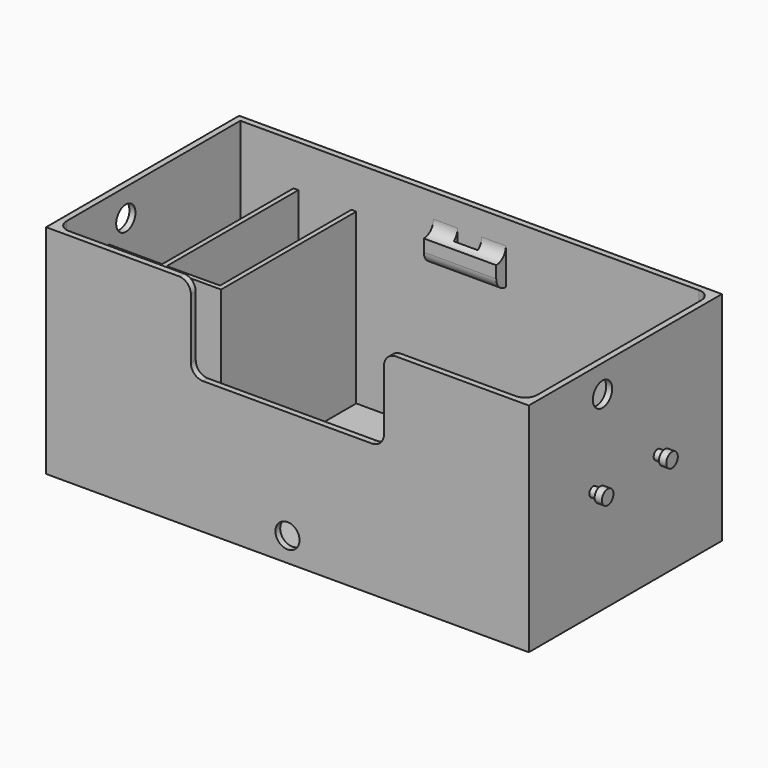
from build123d import *

# Parameters (mm, degrees)
F0_W          = 200
F0_H          = 100
F1_DEPTH      = 90
F2_T          = -2.5
F4_DEPTH      = 70
F5_W          = 80
F5_H          = 35
F5_R          = 5
F6_DEPTH      = 3
F8_DEPTH      = 3
F9_R          = 3.3
F10_DEPTH     = 1.5
F11_R         = 7.8
F12_DEPTH     = 3
F13_R         = 5
F14_R         = 5
F16_DEPTH     = 3
F17_R         = 2
F17_R_2       = 3
F18_R         = 3
F18_R_2       = 2
F19_DEPTH     = 3
F21_DEPTH     = 3
F22_R         = 3
F22_R_2       = 2
F23_DEPTH     = 3
F24_R         = 5
F25_DEPTH     = 400
F26_W         = 22
F26_H         = 30
F26_H_2       = 6.5
F27_W         = 21.9996754151
F27_H         = 30
F29_DEPTH     = 10
F31_W         = 15
F31_H         = 10
F32_DEPTH     = 5
F33_W         = 10
F33_H         = 2
F34_DEPTH     = 10
F35_T4_DEPTH  = 10
F35_T9_DEPTH  = 10
F35_T14_DEPTH = 22.5
F35_T21_DEPTH = 22.5
F35_T27_DEPTH = 22.5
F35_T33_DEPTH = 22.5
F35_T39_DEPTH = 22.5
F35_T45_DEPTH = 22.5
F35_T52_DEPTH = 10
F35_T57_DEPTH = 10
F35_T59_DEPTH = 55
F36_DEPTH     = 35


# Not quite as in the source:
# - a fillet or chamfer that OpenCascade refuses, or shapes differently, is made with other operations: its cross-section is extruded or revolved along the edge and cut away or added
# - ends of sketch curves that miss each other by under 0.0002 mm in the source are joined
# - a feature names something its author has since deleted; it is built from what else it names


with BuildPart() as f1:
    # F0 (on Top) → F1 (new body)
    with BuildSketch(Plane.XY):
        with Locations((-6.9181565195, -17.9440884142)):
            Rectangle(F0_W, F0_H)
    extrude(amount=F1_DEPTH)

    # F2
    f2_openings = [f1.faces().sort_by_distance(p)[0] for p in [
        (-6.918157, -17.944088, 90),
    ]]
    offset(amount=F2_T, openings=f2_openings)

    # F3 (on face) → F4 (join)
    with BuildSketch(Plane.XY.offset(2.5)):
        Polygon((-82.4181565195, -38.4440884142), (-104.4181565195, -38.4440884142), (-104.4181565195, -40.4440884142), (-82.4181565195, -40.4440884142), (-80.4181565195, -40.4440884142), (-80.4181565195, -38.6240089446), (-80.4181565195, 29.5559115858), (-82.4181565195, 29.5559115858), align=None)
        Polygon((-58.4188922454, -38.4440884142), (-80.4181565195, -38.6240089446), (-80.4181565195, -40.4440884142), (-56.4181565195, -40.4440884142), (-56.4181565195, -38.4440884142), (-56.4181565195, 29.5559115858), (-58.4181565195, 29.5559115858), align=None)
    extrude(amount=F4_DEPTH)

    # F5 (on face) → F6 (cut)
    with BuildSketch(Plane.XZ.offset(67.9440884142)):
        with Locations((-6.9181565195, 72.5)):
            Rectangle(F5_W, F5_H)
        with Locations((-6.9181565195, 10)):
            Circle(F5_R)
    extrude(amount=-F6_DEPTH, mode=Mode.SUBTRACT)

    # F7 (on face) → F8 (cut)
    with BuildSketch(Plane(origin=(0, 0, 0), x_dir=(1, 0, 0), z_dir=(0, 0, -1))):
        with BuildLine():
            ThreePointArc((-3.6181565195, 17.9440884142), (-4.5847041416, 20.2775407921), (-6.9181565195, 21.2440884142))
            Line((-6.9181565195, 21.2440884142), (-6.9181565195, 14.6440884142))
            ThreePointArc((-6.9181565195, 14.6440884142), (-4.5847041416, 15.6106360363), (-3.6181565195, 17.9440884142))
        make_face()
        with BuildLine():
            Line((-6.9181565195, 14.6440884142), (-6.9181565195, 21.2440884142))
            ThreePointArc((-6.9181565195, 21.2440884142), (-10.2181565195, 17.9440884142), (-6.9181565195, 14.6440884142))
        make_face()
    extrude(amount=-F8_DEPTH, mode=Mode.SUBTRACT)

    # F9 (on face) → F10 (cut)
    with BuildSketch(Plane.XY.offset(2.5)):
        Polygon((-4.1346192375, -12.3481595191), (-10.3726044595, -12.735509968), (-13.1561417415, -18.3314388632), (-9.7016938016, -23.5400173094), (-3.4637085796, -23.1526668604), (-0.6801712975, -17.5567379653), align=None)
        with Locations((-6.9181565195, -17.9440884142)):
            Circle(F9_R, mode=Mode.SUBTRACT)
    extrude(amount=-F10_DEPTH, mode=Mode.SUBTRACT)

    # F11 (on face) → F12 (cut)
    with BuildSketch(Plane(origin=(0, 32.0559115858, 0), x_dir=(-1, 0, 0), z_dir=(0, 1, 0))):
        with Locations((6.9181565195, 18.6942107975)):
            Circle(F11_R)
    extrude(amount=-F12_DEPTH, mode=Mode.SUBTRACT)

    # F13
    f13_edges = [f1.edges().sort_by_distance(p)[0] for p in [
        (90.581843, 29.555912, 46.25),
        (90.581843, -65.444088, 46.25),
        (-104.418157, -65.444088, 46.25),
    ]]
    fillet(f13_edges, radius=F13_R)

    # F14
    f14_edges = [f1.edges().sort_by_distance(p)[0] for p in [
        (33.081843, -66.694088, 55),
        (-46.918157, -66.694088, 55),
        (-46.918157, -66.694088, 90),
        (33.081843, -66.694088, 90),
    ]]
    fillet(f14_edges, radius=F14_R)

    # F15 (on face) → F16 (join)
    with BuildSketch(Plane.YZ.offset(93.0818434805)):
        with BuildLine():
            ThreePointArc((-32.6107550809, 45), (-34.6107550809, 47), (-36.6107550809, 45))
            Line((-36.6107550809, 45), (-34.6107550809, 45))
            Line((-34.6107550809, 45), (-32.6107550809, 45))
        make_face()
        with BuildLine():
            ThreePointArc((0.7225782525, 45), (-1.2774217475, 47), (-3.2774217475, 45))
            Line((-3.2774217475, 45), (-1.2774217475, 45))
            Line((-1.2774217475, 45), (0.7225782525, 45))
        make_face()
        with BuildLine():
            Line((-1.2774217475, 45), (-3.2774217475, 45))
            ThreePointArc((-3.2774217475, 45), (-1.2774217475, 43), (0.7225782525, 45))
            Line((0.7225782525, 45), (-1.2774217475, 45))
        make_face()
        with BuildLine():
            Line((-34.6107550809, 45), (-36.6107550809, 45))
            ThreePointArc((-36.6107550809, 45), (-34.6107550809, 43), (-32.6107550809, 45))
            Line((-32.6107550809, 45), (-34.6107550809, 45))
        make_face()
    extrude(amount=F16_DEPTH)

    # F17 (on face) + F18 (on face) → F19 (join)
    with BuildSketch(Plane.YZ.offset(96.0818434805)):
        with Locations((-34.6107550809, 45)):
            Circle(F17_R)
        with Locations((-1.2774217475, 45)):
            Circle(F17_R_2)
    with BuildSketch(Plane.YZ.offset(96.0818434805)):
        with Locations((-34.6107550809, 45)):
            Circle(F18_R)
        with Locations((-34.6107550809, 45)):
            Circle(F18_R_2, mode=Mode.SUBTRACT)
    extrude(amount=F19_DEPTH)

    # F20 (on face) → F21 (join)
    with BuildSketch(Plane(origin=(-106.9181565195, 0, 0), x_dir=(0, -1, 0), z_dir=(-1, 0, 0))):
        with BuildLine():
            ThreePointArc((3.2774217475, 45), (1.2774217475, 47), (-0.7225782525, 45))
            Line((-0.7225782525, 45), (1.2774217475, 45))
            Line((1.2774217475, 45), (3.2774217475, 45))
        make_face()
        with BuildLine():
            Line((1.2774217475, 45), (-0.7225782525, 45))
            ThreePointArc((-0.7225782525, 45), (1.2774217475, 43), (3.2774217475, 45))
            Line((3.2774217475, 45), (1.2774217475, 45))
        make_face()
        with BuildLine():
            ThreePointArc((36.6107550809, 45), (34.6107550809, 47), (32.6107550809, 45))
            Line((32.6107550809, 45), (34.6107550809, 45))
            Line((34.6107550809, 45), (36.6107550809, 45))
        make_face()
        with BuildLine():
            Line((34.6107550809, 45), (32.6107550809, 45))
            ThreePointArc((32.6107550809, 45), (34.6107550809, 43), (36.6107550809, 45))
            Line((36.6107550809, 45), (34.6107550809, 45))
        make_face()
    extrude(amount=F21_DEPTH)

    # F22 (on face) → F23 (join)
    with BuildSketch(Plane(origin=(-109.9181565195, 0, 0), x_dir=(0, -1, 0), z_dir=(-1, 0, 0))):
        with Locations((1.2774217475, 45)):
            Circle(F22_R)
        with Locations((1.2774217475, 45)):
            Circle(F22_R_2, mode=Mode.SUBTRACT)
        with Locations((1.2774217475, 45)):
            Circle(F22_R_2)
        with Locations((34.6107550809, 45)):
            Circle(F22_R)
    extrude(amount=F23_DEPTH)

    # F24 (on face) → F25 (cut, symmetric)
    with BuildSketch(Plane.YZ.offset(-104.4181565195)):
        with Locations((-29.7736749053, 78.6124244332)):
            Circle(F24_R)
    extrude(amount=F25_DEPTH, both=True, mode=Mode.SUBTRACT)

    # F26 (on face) + F27 (on face) + F28 (on face) → F29 (join)
    with BuildSketch(Plane.XY.offset(2.5)):
        with Locations((-93.4181565195, 14.5559115858)):
            Rectangle(F26_W, F26_H)
        with Locations((-93.4181565195, -35.1940884142)):
            Rectangle(F26_W, F26_H_2)
    with BuildSketch(Plane.XY.offset(2.5)):
        with Locations((-69.418318812, 14.5559115858)):
            Rectangle(F27_W, F27_H)
        Polygon((-58.4181565195, 29.5559115858), (-58.4184811045, 29.5559115858), (-58.4184811045, -0.4440884142), align=None)
    with BuildSketch(Plane.XY.offset(2.5)):
        Polygon((-80.4181565195, -32.1240089446), (-80.4181565195, -38.6240089446), (-58.4188922454, -38.4440884142), (-58.4188238653, -32.1240089446), align=None)
    extrude(amount=F29_DEPTH)

    # F31 (on face) → F32 (join)
    with BuildSketch(Plane.XZ.offset(-29.5559115858)):
        with Locations((-16.9181565195, 70.1089176536)):
            Rectangle(F31_W, F31_H)
        with Locations((-1.9181565195, 70.1089176536)):
            Rectangle(F31_W, F31_H)
    extrude(amount=F32_DEPTH)

    # F33 (on face) → F34 (cut)
    with BuildSketch(Plane.XY.offset(75.1089176536)):
        with Locations((-9.4181565195, 28.5559115858)):
            Rectangle(F33_W, F33_H)
    extrude(amount=-F34_DEPTH, mode=Mode.SUBTRACT)

    # F35: fillet of radius 5 on 3 edges, made by hand


with BuildPart() as f35_tool2:
    # F35_s3 → F35_t4 (new body)
    with BuildSketch(Plane.YZ.offset(5.5818434805)):
        with BuildLine():
            ThreePointArc((29.5559115858, 80.1089176536), (28.0914454917, 76.5733837476), (24.5559115858, 75.1089176536))
            Line((24.5559115858, 75.1089176536), (29.5559115858, 75.1089176536))
            Line((29.5559115858, 75.1089176536), (29.5559115858, 80.1089176536))
        make_face()
    extrude(amount=-F35_T4_DEPTH)

    split(bisect_by=Plane.XZ.offset(-27.5559115858), keep=Keep.BOTTOM)


with BuildPart() as f1_1:
    add(f1.part)

    # F35_t1: union F35_tool2
    add(f35_tool2.part)


with BuildPart() as f35_tool7:
    # F35_s8 → F35_t9 (new body)
    with BuildSketch(Plane.YZ.offset(5.5818434805)):
        with BuildLine():
            ThreePointArc((29.5559115858, 80.1089176536), (28.0914454917, 76.5733837476), (24.5559115858, 75.1089176536))
            Line((24.5559115858, 75.1089176536), (29.5559115858, 75.1089176536))
            Line((29.5559115858, 75.1089176536), (29.5559115858, 80.1089176536))
        make_face()
    extrude(amount=-F35_T9_DEPTH)

    split(bisect_by=Plane.XZ.offset(-27.5559115858), keep=Keep.TOP)


with BuildPart() as f1_2:
    add(f1_1.part)

    # F35_t6: union F35_tool7
    add(f35_tool7.part)


with BuildPart() as f35_tool12:
    # F35_s13 → F35_t14 (new body)
    with BuildSketch(Plane.YZ.offset(5.5818434805)):
        with BuildLine():
            ThreePointArc((29.5559115858, 80.1089176536), (28.0914454917, 76.5733837476), (24.5559115858, 75.1089176536))
            Line((24.5559115858, 75.1089176536), (29.5559115858, 75.1089176536))
            Line((29.5559115858, 75.1089176536), (29.5559115858, 80.1089176536))
        make_face()
    extrude(amount=-F35_T14_DEPTH)

    split(bisect_by=Plane.YZ.offset(-4.4181565195), keep=Keep.BOTTOM)

    split(bisect_by=Plane.XZ.offset(-27.5559115858), keep=Keep.TOP)

    split(bisect_by=Plane.YZ.offset(-14.4181565195), keep=Keep.TOP)


with BuildPart() as f1_3:
    add(f1_2.part)

    # F35_t11: union F35_tool12
    add(f35_tool12.part)


with BuildPart() as f35_tool19:
    # F35_s20 → F35_t21 (new body)
    with BuildSketch(Plane.YZ.offset(5.5818434805)):
        with BuildLine():
            ThreePointArc((29.5559115858, 80.1089176536), (28.0914454917, 76.5733837476), (24.5559115858, 75.1089176536))
            Line((24.5559115858, 75.1089176536), (29.5559115858, 75.1089176536))
            Line((29.5559115858, 75.1089176536), (29.5559115858, 80.1089176536))
        make_face()
    extrude(amount=-F35_T21_DEPTH)

    split(bisect_by=Plane.XZ.offset(-27.5559115858), keep=Keep.BOTTOM)

    split(bisect_by=Plane.YZ.offset(-14.4181565195), keep=Keep.BOTTOM)


with BuildPart() as f1_4:
    add(f1_3.part)

    # F35_t18: union F35_tool19
    add(f35_tool19.part)


with BuildPart() as f35_tool25:
    # F35_s26 → F35_t27 (new body)
    with BuildSketch(Plane.YZ.offset(5.5818434805)):
        with BuildLine():
            ThreePointArc((29.5559115858, 80.1089176536), (28.0914454917, 76.5733837476), (24.5559115858, 75.1089176536))
            Line((24.5559115858, 75.1089176536), (29.5559115858, 75.1089176536))
            Line((29.5559115858, 75.1089176536), (29.5559115858, 80.1089176536))
        make_face()
    extrude(amount=-F35_T27_DEPTH)

    split(bisect_by=Plane.XZ.offset(-27.5559115858), keep=Keep.TOP)

    split(bisect_by=Plane.YZ.offset(-14.4181565195), keep=Keep.BOTTOM)


with BuildPart() as f1_5:
    add(f1_4.part)

    # F35_t24: union F35_tool25
    add(f35_tool25.part)


with BuildPart() as f35_tool31:
    # F35_s32 → F35_t33 (new body)
    with BuildSketch(Plane.YZ.offset(-1.9181565195)):
        with BuildLine():
            ThreePointArc((29.5559115858, 80.1089176536), (28.0914454917, 76.5733837476), (24.5559115858, 75.1089176536))
            Line((24.5559115858, 75.1089176536), (29.5559115858, 75.1089176536))
            Line((29.5559115858, 75.1089176536), (29.5559115858, 80.1089176536))
        make_face()
    extrude(amount=-F35_T33_DEPTH)

    split(bisect_by=Plane.YZ.offset(-4.4181565195), keep=Keep.TOP)

    split(bisect_by=Plane.XZ.offset(-27.5559115858), keep=Keep.BOTTOM)


with BuildPart() as f1_6:
    add(f1_5.part)

    # F35_t30: union F35_tool31
    add(f35_tool31.part)


with BuildPart() as f35_tool37:
    # F35_s38 → F35_t39 (new body)
    with BuildSketch(Plane.YZ.offset(-1.9181565195)):
        with BuildLine():
            ThreePointArc((29.5559115858, 80.1089176536), (28.0914454917, 76.5733837476), (24.5559115858, 75.1089176536))
            Line((24.5559115858, 75.1089176536), (29.5559115858, 75.1089176536))
            Line((29.5559115858, 75.1089176536), (29.5559115858, 80.1089176536))
        make_face()
    extrude(amount=-F35_T39_DEPTH)

    split(bisect_by=Plane.YZ.offset(-4.4181565195), keep=Keep.TOP)

    split(bisect_by=Plane.XZ.offset(-27.5559115858), keep=Keep.TOP)


with BuildPart() as f1_7:
    add(f1_6.part)

    # F35_t36: union F35_tool37
    add(f35_tool37.part)


with BuildPart() as f35_tool43:
    # F35_s44 → F35_t45 (new body)
    with BuildSketch(Plane.YZ.offset(-1.9181565195)):
        with BuildLine():
            ThreePointArc((29.5559115858, 80.1089176536), (28.0914454917, 76.5733837476), (24.5559115858, 75.1089176536))
            Line((24.5559115858, 75.1089176536), (29.5559115858, 75.1089176536))
            Line((29.5559115858, 75.1089176536), (29.5559115858, 80.1089176536))
        make_face()
    extrude(amount=-F35_T45_DEPTH)

    split(bisect_by=Plane.YZ.offset(-14.4181565195), keep=Keep.TOP)

    split(bisect_by=Plane.YZ.offset(-4.4181565195), keep=Keep.BOTTOM)

    split(bisect_by=Plane.XZ.offset(-27.5559115858), keep=Keep.TOP)


with BuildPart() as f1_8:
    add(f1_7.part)

    # F35_t42: union F35_tool43
    add(f35_tool43.part)


with BuildPart() as f35_tool50:
    # F35_s51 → F35_t52 (new body)
    with BuildSketch(Plane.YZ.offset(-14.4181565195)):
        with BuildLine():
            ThreePointArc((29.5559115858, 80.1089176536), (28.0914454917, 76.5733837476), (24.5559115858, 75.1089176536))
            Line((24.5559115858, 75.1089176536), (29.5559115858, 75.1089176536))
            Line((29.5559115858, 75.1089176536), (29.5559115858, 80.1089176536))
        make_face()
    extrude(amount=-F35_T52_DEPTH)

    split(bisect_by=Plane.XZ.offset(-27.5559115858), keep=Keep.BOTTOM)


with BuildPart() as f1_9:
    add(f1_8.part)

    # F35_t49: union F35_tool50
    add(f35_tool50.part)


with BuildPart() as f35_tool55:
    # F35_s56 → F35_t57 (new body)
    with BuildSketch(Plane.YZ.offset(-14.4181565195)):
        with BuildLine():
            ThreePointArc((29.5559115858, 80.1089176536), (28.0914454917, 76.5733837476), (24.5559115858, 75.1089176536))
            Line((24.5559115858, 75.1089176536), (29.5559115858, 75.1089176536))
            Line((29.5559115858, 75.1089176536), (29.5559115858, 80.1089176536))
        make_face()
    extrude(amount=-F35_T57_DEPTH)

    split(bisect_by=Plane.XZ.offset(-27.5559115858), keep=Keep.TOP)


with BuildPart() as f1_10:
    add(f1_9.part)

    # F35_t54: union F35_tool55
    add(f35_tool55.part)

    # F35_s60 → F35_t59 (cut)
    with BuildSketch(Plane.YZ.offset(-36.9181565195)):
        with BuildLine():
            ThreePointArc((24.5559115858, 70.1089176536), (26.0203776799, 66.5733837476), (29.5559115858, 65.1089176536))
            Line((29.5559115858, 65.1089176536), (24.5559115858, 65.1089176536))
            Line((24.5559115858, 65.1089176536), (24.5559115858, 70.1089176536))
        make_face()
    extrude(amount=F35_T59_DEPTH, mode=Mode.SUBTRACT)

    # F30 (on face) → F36 (cut)
    with BuildSketch(Plane.YZ.offset(-56.4181565195)):
        with BuildLine():
            ThreePointArc((-30.4440884142, 4.5), (-27.3464061616, 3.113491758), (-25.2552007889, 5.786486433))
            ThreePointArc((-25.2552007889, 5.786486433), (-28.6718429924, 8.459481108), (-30.4440884142, 4.5))
        make_face()
    extrude(amount=-F36_DEPTH, mode=Mode.SUBTRACT)


solid = f1_10.part
